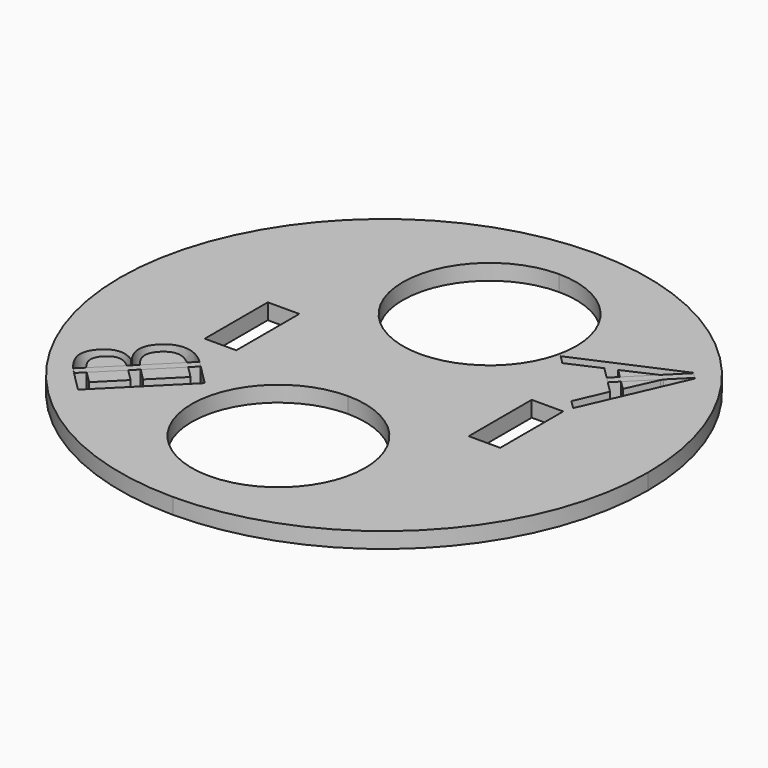
from build123d import *

# Parameters (mm, degrees)
F2_DEPTH     = 2
F3_TEXT_SIZE = 17.7066410995
F4_DEPTH     = 25
F6_DEPTH     = 2


# Not quite as in the source:
# - Text() gives the source's letters only with a copy of the font that has no kerning and outlines rounded to 1/6400 em; it was checked with that copy


with BuildPart() as f2:
    # F1 (on Top) → F2 (new body)
    with BuildSketch(Plane.XY):
        with BuildLine():
            ThreePointArc((-33.5, 0), (-23.6880771697, -23.6880771697), (0, -33.5))
            Line((0, -33.5), (0, -27.75))
            ThreePointArc((0, -27.75), (-11, -16.75), (0, -5.75))
            Line((0, -5.75), (0, 0))
            Line((0, 0), (-14.75, 0))
            Line((-14.75, 0), (-14.75, -5))
            Line((-14.75, -5), (-18.75, -5))
            Line((-18.75, -5), (-18.75, 0))
            Line((-18.75, 0), (-33.5, 0))
        make_face()
        with BuildLine():
            Line((0, 27.75), (0, 33.5))
            ThreePointArc((0, 33.5), (-23.6880771697, 23.6880771697), (-33.5, 0))
            Line((-33.5, 0), (-18.75, 0))
            Line((-18.75, 0), (-18.75, 5))
            Line((-18.75, 5), (-14.75, 5))
            Line((-14.75, 5), (-14.75, 0))
            Line((-14.75, 0), (0, 0))
            Line((0, 0), (0, 5.75))
            ThreePointArc((0, 5.75), (-11, 16.75), (0, 27.75))
        make_face()
        with BuildLine():
            Line((18.75, 0), (33.5, 0))
            ThreePointArc((33.5, 0), (23.6880771697, 23.6880771697), (0, 33.5))
            Line((0, 33.5), (0, 27.75))
            ThreePointArc((0, 27.75), (7.7781745931, 24.5281745931), (11, 16.75))
            ThreePointArc((11, 16.75), (7.7781745931, 8.9718254069), (0, 5.75))
            Line((0, 5.75), (0, 0))
            Line((0, 0), (14.75, 0))
            Line((14.75, 0), (14.75, 5))
            Line((14.75, 5), (18.75, 5))
            Line((18.75, 5), (18.75, 0))
        make_face()
        with BuildLine():
            ThreePointArc((0, -33.5), (23.6880771697, -23.6880771697), (33.5, 0))
            Line((33.5, 0), (18.75, 0))
            Line((18.75, 0), (18.75, -5))
            Line((18.75, -5), (14.75, -5))
            Line((14.75, -5), (14.75, 0))
            Line((14.75, 0), (0, 0))
            Line((0, 0), (0, -5.75))
            ThreePointArc((0, -5.75), (7.7781745931, -8.9718254069), (11, -16.75))
            ThreePointArc((11, -16.75), (7.7781745931, -24.5281745931), (0, -27.75))
            Line((0, -27.75), (0, -33.5))
        make_face()
    extrude(amount=F2_DEPTH)

    # F3 (on face) → F4 (cut)
    with BuildSketch(Plane.XY.offset(2)):
        with Locations(Location((-11.5607743401, -13.6805723544), (0, 0, 135))):
            Text('B', F3_TEXT_SIZE, font='Open Sans', text_align=(TextAlign.LEFT, TextAlign.BOTTOM))
        with Locations(Location((11.1475059822, 14.0947057627), (0, 0, -45))):
            Text('A', F3_TEXT_SIZE, font='Open Sans', text_align=(TextAlign.LEFT, TextAlign.BOTTOM))
    extrude(amount=-F4_DEPTH, mode=Mode.SUBTRACT)


with BuildPart() as f6:
    # F5 (on face) → F6 (new body)
    with BuildSketch(Plane.XY.offset(2)):
        Polygon((18.2865758835, 12.6407190328), (24.4196576944, 18.7738008437), (23.7125509132, 19.4809076249), (17.5794691024, 13.347825814), align=None)
    extrude(amount=-F6_DEPTH)


with BuildPart() as f6b:
    # F5 (on face) → F6, piece 2 (new body)
    with BuildSketch(Plane.XY.offset(2)):
        with BuildLine():
            Line((-16.0423016256, -9.201918939), (-24.9542306343, -18.1138479476))
            add(Edge.make_bspline(
                [(-24.9542306343, -18.1138479476), (-24.6472106734, -18.469819549), (-24.2721962109, -18.8460270866)],
                knots=[4.5713616302, 4.5713616302, 4.5713616302, 4.8768884025, 4.8768884025, 4.8768884025], degree=2))
            Line((-24.2721962109, -18.8460270866), (-15.3337579094, -9.9075887851))
            Line((-15.3337579094, -9.9075887851), (-15.907730571, -9.3336161236))
            add(Edge.make_bspline(
                [(-15.907730571, -9.3336161236), (-15.9749868583, -9.2663598362), (-16.0423016256, -9.201918939)],
                knots=[0, 0, 0, 0.0462081671, 0.0462081671, 0.0462081671], degree=2))
        make_face()
    extrude(amount=-F6_DEPTH)


solid = Compound([f2.part, f6.part, f6b.part])
